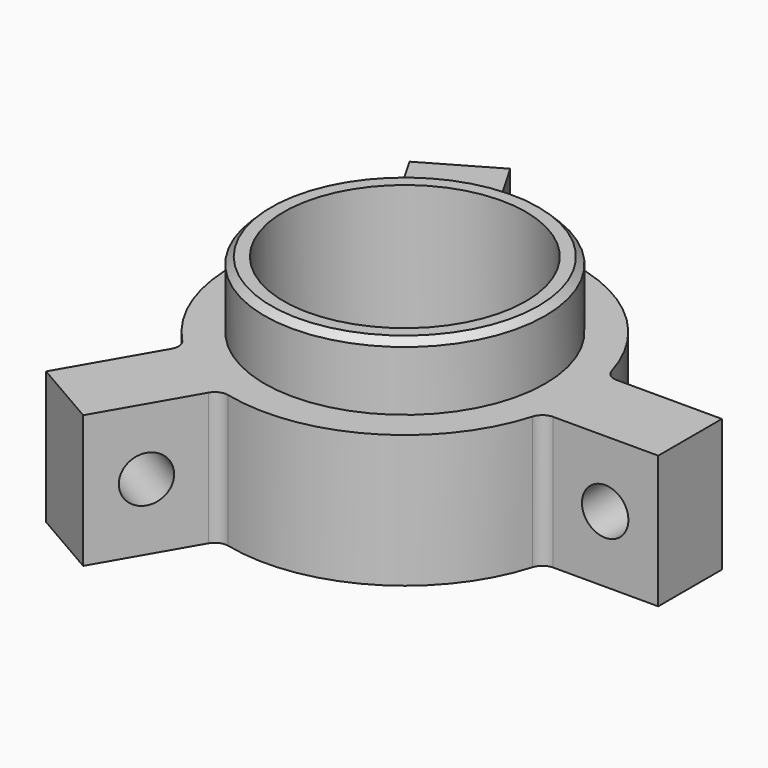
from build123d import *

# Parameters (mm, degrees)
F2_W            = 43
F2_H            = 20
F2_R            = 3.5
F3_DEPTH        = 6
F3_COPIES_COUNT = 3
F4_R            = 18.25
F5_DEPTH        = 30.001
F6_SIZE         = 1
F7_R            = 2


# Not quite as in the source:
# - a pattern or mirror of a feature is missing from the dataset's text; its kind, count and spacing are read off the source's solid


with BuildPart() as f1:
    # F0 (on Front) → F1 (revolve)
    with BuildSketch(Plane.XZ):
        Polygon((21.15, 30), (0, 30), (0, 0), (26.3, 0), (26.3, 20), (21.15, 20), align=None)
    revolve(axis=Axis((0, 0, 22.5), (0, 0, 1)))

    # F2 (on Front) → F3 (join, symmetric)
    with BuildSketch(Plane.XZ):
        with Locations((21.5, 10)):
            Rectangle(F2_W, F2_H)
        with Locations((35, 10)):
            Circle(F2_R, mode=Mode.SUBTRACT)
    f3 = extrude(amount=F3_DEPTH, both=True)

    # F3_copies: F3 ×3 about axis
    f3_copies_axis = Axis((0, 0, 0), (0, 0, 1))
    for i in range(1, F3_COPIES_COUNT):
        add(f3.rotate(f3_copies_axis, i * 360 / F3_COPIES_COUNT))

    # F4 (on Top) → F5 (cut, through all)
    with BuildSketch(Plane.XY):
        Circle(F4_R)
    extrude(amount=F5_DEPTH, mode=Mode.SUBTRACT)

    # F6
    f6_edges = [f1.edges().sort_by_distance(p)[0] for p in [
        (-21.15, 0, 30),
    ]]
    chamfer(f6_edges, length=F6_SIZE)

    # F7
    f7_edges = [f1.edges().sort_by_distance(p)[0] for p in [
        (25.606445, -6, 10),
        (25.606445, 6, 10),
        (-7.60707, 25.175831, 10),
        (-17.999375, 19.175831, 10),
        (-7.60707, -25.175831, 10),
        (-17.999375, -19.175831, 10),
    ]]
    fillet(f7_edges, radius=F7_R)


solid = f1.part
